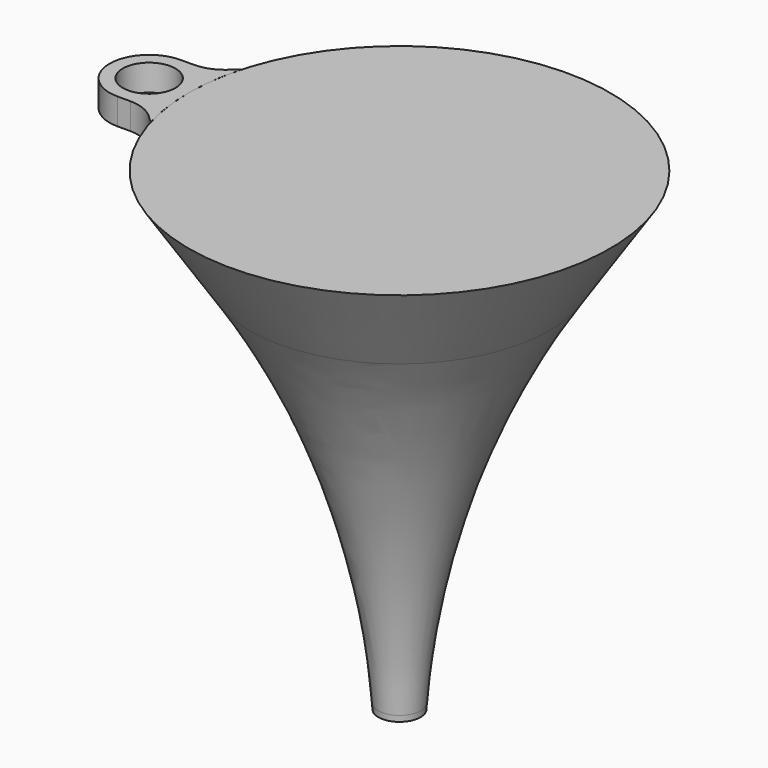
from build123d import *

# Parameters (mm, degrees)
F2_R        = 150
F3_R        = 5
F4_DEPTH    = 5
F6_T1_DEPTH = 25.7103664143


# Not quite as in the source:
# - a fillet or chamfer that OpenCascade refuses, or shapes differently, is made with other operations: its cross-section is extruded or revolved along the edge and cut away or added


with BuildPart() as f1:
    # F0 (on Front) → F1 (revolve)
    with BuildSketch(Plane.XZ):
        Polygon((-7, 40), (-4, 0), (0, 0), (0, 90), (-40, 90), align=None)
    revolve(axis=Axis((0, 0, 45), (0, 0, -1)))

    # F2
    f2_edges = [f1.edges().sort_by_distance(p)[0] for p in [
        (7, 0, 40),
    ]]
    fillet(f2_edges, radius=F2_R)


with BuildPart() as f4:
    # F3 (on face) → F4 (new body)
    with BuildSketch(Plane.XY.offset(90)):
        with BuildLine():
            Line((-45.0693909433, 7.5), (-47.5, 7.5))
            ThreePointArc((-47.5, 7.5), (-52.8033008589, 5.3033008589), (-55, 0))
            ThreePointArc((-55, 0), (-52.8033008589, -5.3033008589), (-47.5, -7.5))
            Line((-47.5, -7.5), (-45.0693909433, -7.5))
            ThreePointArc((-45.0693909433, -7.5), (-40.6826585543, -8.9166967076), (-37.9531713207, -12.6315789474))
            ThreePointArc((-37.9531713207, -12.6315789474), (-38.707011174, -10.0879772984), (-39.2905841138, -7.5))
            ThreePointArc((-39.2905841138, -7.5), (-40, 0), (-39.2905841138, 7.5))
            ThreePointArc((-39.2905841138, 7.5), (-38.707011174, 10.0879772984), (-37.9531713207, 12.6315789474))
            ThreePointArc((-37.9531713207, 12.6315789474), (-40.6826585543, 8.9166967076), (-45.0693909433, 7.5))
        make_face()
        with Locations((-47.5, 0)):
            Circle(F3_R, mode=Mode.SUBTRACT)
        with BuildLine():
            Line((-25, 7.5), (-37.9531713207, 12.6315789474))
            ThreePointArc((-37.9531713207, 12.6315789474), (-38.707011174, 10.0879772984), (-39.2905841138, 7.5))
            ThreePointArc((-39.2905841138, 7.5), (-40, 0), (-39.2905841138, -7.5))
            ThreePointArc((-39.2905841138, -7.5), (-38.707011174, -10.0879772984), (-37.9531713207, -12.6315789474))
            Line((-37.9531713207, -12.6315789474), (-25, -7.5))
            Line((-25, -7.5), (-25, 7.5))
        make_face()
    extrude(amount=-F4_DEPTH)

    # F0 (on Front) → F5 (revolve, cut)
    with BuildSketch(Plane.XZ):
        Polygon((-7, 40), (-4, 0), (0, 0), (0, 90), (-40, 90), align=None)
    revolve(axis=Axis((0, 0, 45), (0, 0, -1)), mode=Mode.SUBTRACT)

    # F6: fillet of radius 5 on 2 edges, made by hand

    # F6_s2 → F6_t1 (cut)
    with BuildSketch(Plane.XY.offset(74.6448167928)):
        with BuildLine():
            ThreePointArc((-34.102279986, -11.1059947941), (-37.0379022892, -11.33632485), (-39.5940667848, -9.874492673))
            ThreePointArc((-39.5940667848, -9.874492673), (-38.6244607746, -11.1642634187), (-37.9531713207, -12.6315789474))
            Line((-37.9531713207, -12.6315789474), (-34.102279986, -11.1059947941))
        make_face()
        with BuildLine():
            ThreePointArc((-39.5940667848, 9.874492673), (-37.0379022892, 11.33632485), (-34.102279986, 11.1059947941))
            Line((-34.102279986, 11.1059947941), (-37.9531713207, 12.6315789474))
            ThreePointArc((-37.9531713207, 12.6315789474), (-38.6244607746, 11.1642634187), (-39.5940667848, 9.874492673))
        make_face()
    extrude(amount=F6_T1_DEPTH, mode=Mode.SUBTRACT)


solid = Compound([f1.part, f4.part])
